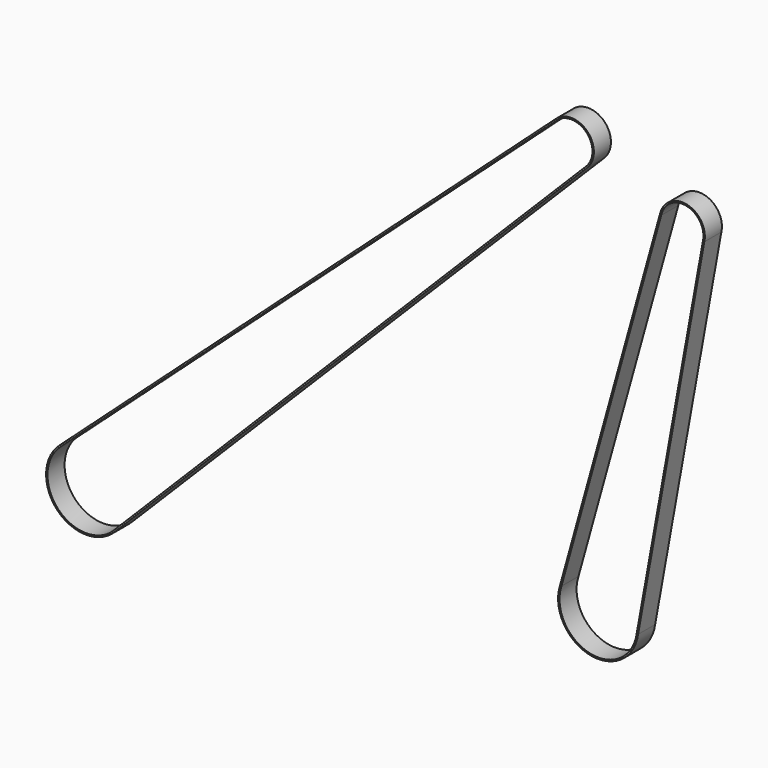
from build123d import *
from build123d import SkipClean  # not in build123d's __all__

# Parameters (mm, degrees)
F1_DEPTH  = 15
F2_R      = 8
F2_R_2    = 3
F3_DEPTH  = 10
F4_R      = 8
F4_R_2    = 3
F5_DEPTH  = 10
F6_R      = 8
F6_R_2    = 3
F7_DEPTH  = 10
F8_R      = 27.25
F8_R_2    = 15
F9_DEPTH  = 20
F11_R     = 15
F11_R_2   = 27.25
F12_DEPTH = 20


with BuildPart() as f1:
    # F0 (on Front) → F1 (new body)
    with BuildSketch(Plane.XZ):
        with BuildLine():
            ThreePointArc((-378.4425772317, 201.3993888944), (-386.4820244342, 170.1630857548), (-360, 151.75))
            ThreePointArc((-360, 151.75), (-348.8330724465, 154.0507759458), (-339.4850899056, 160.5783377689))
            Line((-339.4850899056, 160.5783377689), (-7.9870573254, 493.2915694615))
            ThreePointArc((-7.9870573254, 493.2915694615), (-7.480425283, 515.8738544687), (-30.0608082206, 516.4591565815))
            Line((-30.0608082206, 516.4591565815), (-378.4425772317, 201.3993888944))
        make_face()
        with BuildLine():
            ThreePointArc((-342.5, 180), (-347.6256313292, 167.6256313292), (-360, 162.5))
            ThreePointArc((-360, 162.5), (-376.0857600208, 186.8919028253), (-347.3301148646, 192.071620051))
            ThreePointArc((-347.3301148646, 192.071620051), (-343.7523387857, 186.5010387682), (-342.5, 180))
        make_face(mode=Mode.SUBTRACT)
        with BuildLine():
            ThreePointArc((-340.2025834833, 161.275022049), (-332.7500455353, 180.0498163798), (-340.2711788606, 198.7972369366))
            ThreePointArc((-340.2711788606, 198.7972369366), (-358.6559201587, 207.2168320967), (-377.7807722421, 200.6496159401))
            Line((-377.7807722421, 200.6496159401), (-29.3815729723, 515.7251467174))
            ThreePointArc((-29.3815729723, 515.7251467174), (-34.059394529, 505.2200757083), (-29.9241906854, 494.4898091415))
            ThreePointArc((-29.9241906854, 494.4898091415), (-19.406287314, 489.8408113075), (-8.6873810185, 494.0054865673))
            Line((-8.6873810185, 494.0054865673), (-340.2025834833, 161.275022049))
        make_face(mode=Mode.SUBTRACT)
        with BuildLine():
            ThreePointArc((-16.0642891408, 504.8369120424), (-17.949825352, 502.0515986913), (-21.2362694497, 502.7674914622))
            ThreePointArc((-21.2362694497, 502.7674914622), (-20.1787529296, 507.6222253934), (-16.0642891408, 504.8369120424))
        make_face(mode=Mode.SUBTRACT)
    extrude(amount=F1_DEPTH)

    # F4 (on face) → F5 (join)
    with BuildSketch(Plane.XZ.offset(15)):
        with Locations((-19.0642891408, 504.8369120424)):
            Circle(F4_R)
        with Locations((-19.0642891408, 504.8369120424)):
            Circle(F4_R_2, mode=Mode.SUBTRACT)
    extrude(amount=F5_DEPTH)

    # F11 (on face) → F12 (cut, symmetric)
    with BuildSketch(Plane.XZ.offset(15)):
        with Locations((-19.0642891408, 504.8369120424)):
            Circle(F11_R)
        with Locations((-360, 180)):
            Circle(F11_R_2)
    with SkipClean():  # cleaning this boolean's faces spoils the solid; the shape is the same uncleaned
        extrude(amount=F12_DEPTH, both=True, mode=Mode.SUBTRACT)


with BuildPart() as f1b:
    # F0 (on Front) → F1, piece 2 (new body)
    with BuildSketch(Plane.XZ):
        with BuildLine():
            ThreePointArc((-224.660632779, 532.8994691874), (-247.0029596883, 497.3937658802), (-209.3929270309, 478.8109786144))
            Line((-209.3929270309, 478.8109786144), (4.2800251225, 551.6775062268))
            ThreePointArc((4.2800251225, 551.6775062268), (15.2214539509, 571.3907533569), (-4.4127934903, 582.4733209582))
            Line((-4.4127934903, 582.4733209582), (-224.660632779, 532.8994691874))
        make_face()
        with BuildLine():
            ThreePointArc((-202.3153298886, 505.0680922919), (-237.1501331245, 502.669218229), (-202.9729980908, 509.8205505625))
            ThreePointArc((-202.9729980908, 509.8205505625), (-202.4805266526, 507.4669663547), (-202.3153298886, 505.0680922919))
        make_face(mode=Mode.SUBTRACT)
        with BuildLine():
            ThreePointArc((-4.1701281966, 581.5029225476), (-13.2448658651, 574.4081273865), (-14.6131340506, 562.9706965429))
            ThreePointArc((-14.6131340506, 562.9706965429), (-7.4667919525, 553.9348179807), (3.9795568505, 552.6315889697))
            Line((3.9795568505, 552.6315889697), (-209.7391973494, 479.7494419911))
            ThreePointArc((-209.7391973494, 479.7494419911), (-195.37987596, 493.0069525734), (-193.589413232, 512.4683487418))
            ThreePointArc((-193.589413232, 512.4683487418), (-205.2909288271, 528.1246374322), (-224.4651790674, 531.9184442936))
            Line((-224.4651790674, 531.9184442936), (-4.1701281966, 581.5029225476))
        make_face(mode=Mode.SUBTRACT)
        with BuildLine():
            ThreePointArc((2.8231503475, 567.0442322034), (0.2343859011, 564.0725516487), (-3.0641065321, 566.2295250713))
            ThreePointArc((-3.0641065321, 566.2295250713), (-0.5880852061, 570.0159127581), (2.8231503475, 567.0442322034))
        make_face(mode=Mode.SUBTRACT)
    extrude(amount=F1_DEPTH)

    # F6 (on face) → F7 (join)
    with BuildSketch(Plane.XZ.offset(15)):
        with Locations((-0.1768496525, 567.0442322034)):
            Circle(F6_R)
        with Locations((-0.1768496525, 567.0442322034)):
            Circle(F6_R_2, mode=Mode.SUBTRACT)
    extrude(amount=F7_DEPTH)


with BuildPart() as f1c:
    # F0 (on Front) → F1, piece 3 (new body)
    with BuildSketch(Plane.XZ):
        with BuildLine():
            ThreePointArc((-26.8437130081, 228.8884241481), (-6.2735642109, 192.6293687538), (28.0157804914, 216.3378263061))
            Line((28.0157804914, 216.3378263061), (74.5878668874, 474.4741693703))
            ThreePointArc((74.5878668874, 474.4741693703), (62.3717320494, 493.5768497593), (43.3204306097, 481.2807421686))
            Line((43.3204306097, 481.2807421686), (-26.8437130081, 228.8884241481))
        make_face()
        with BuildLine():
            ThreePointArc((17.526619941, 220.1678904943), (-13.6575690894, 209.2595005773), (3.9274233032, 237.2276013104))
            ThreePointArc((3.9274233032, 237.2276013104), (13.7108089714, 231.0762804113), (17.526619941, 220.1678904943))
        make_face(mode=Mode.SUBTRACT)
        with BuildLine():
            ThreePointArc((44.2921973879, 481.0427708065), (46.331220076, 469.862073162), (55.6248700068, 463.3203849774))
            ThreePointArc((55.6248700068, 463.3203849774), (66.9752801691, 465.2587472424), (73.607367574, 474.6717422905))
            Line((73.607367574, 474.6717422905), (27.027861197, 216.4942723007))
            ThreePointArc((27.027861197, 216.4942723007), (22.4337443248, 235.6754137282), (6.1007280336, 246.7322973366))
            ThreePointArc((6.1007280336, 246.7322973366), (-13.4116938297, 243.8738860018), (-25.8860157877, 228.5998422013))
            Line((-25.8860157877, 228.5998422013), (44.2921973879, 481.0427708065))
        make_face(mode=Mode.SUBTRACT)
        with BuildLine():
            ThreePointArc((61.9684157458, 477.9429942484), (60.8384254459, 475.5971332717), (58.299706598, 475.0184723942))
            ThreePointArc((58.299706598, 475.0184723942), (57.0984060458, 480.288855225), (61.9684157458, 477.9429942484))
        make_face(mode=Mode.SUBTRACT)
    extrude(amount=F1_DEPTH)

    # F2 (on face) → F3 (join)
    with BuildSketch(Plane.XZ.offset(15)):
        with Locations((58.9684157458, 477.9429942484)):
            Circle(F2_R)
        with Locations((58.9684157458, 477.9429942484)):
            Circle(F2_R_2, mode=Mode.SUBTRACT)
    with SkipClean():  # cleaning this boolean's faces spoils the solid; the shape is the same uncleaned
        extrude(amount=F3_DEPTH)

    # F8 (on face) → F9 (cut, symmetric)
    with BuildSketch(Plane.XZ.offset(15)):
        with Locations((0.026619941, 220.1678904943)):
            Circle(F8_R)
        with Locations((58.9684157458, 477.9429942484)):
            Circle(F8_R_2)
    extrude(amount=F9_DEPTH, both=True, mode=Mode.SUBTRACT)


solid = Compound([f1.part, f1c.part])
